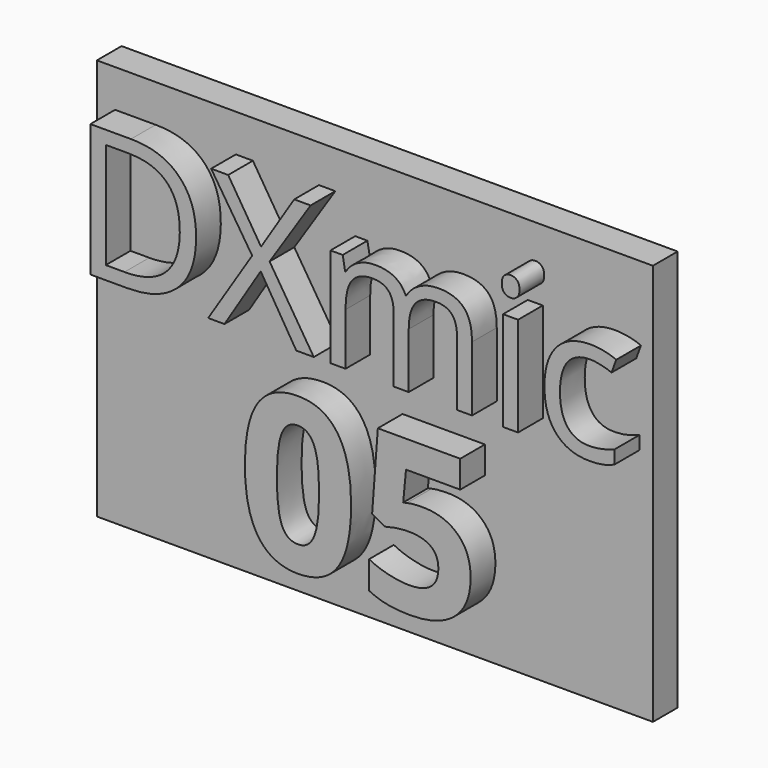
from build123d import *

# Parameters (mm, degrees)
F0_W           = 36
F0_H           = 26
F0_W_2         = 0.9740889422
F0_H_2         = 6.4282362755
F0_TEXT_SIZE   = 13.7795519549
F0_TEXT_SIZE_2 = 12.0118867629
F1_DEPTH       = 2
F2_DEPTH       = 2


# Not quite as in the source:
# - Text() gives the source's letters only with a copy of the font that has no kerning and outlines rounded to 1/6400 em; it was checked with that copy


with BuildPart() as f1:
    # F0 (on Front) → F1 (new body)
    with BuildSketch(Plane.XZ):
        with Locations((-18, 13)):
            Rectangle(F0_W, F0_H)
        with BuildLine():
            add(Edge.make_bspline(
                [(-18.8107192494, 11.141487038), (-17.9398085047, 9.8496540422), (-17.9398085047, 7.3585694154)],
                knots=[0, 0, 0, 1, 1, 1], degree=2))
            add(Edge.make_bspline(
                [(-17.9398085047, 7.3585694154), (-17.9398085047, 4.7835156438), (-18.7838060619, 3.5444324953)],
                knots=[0, 0, 0, 1, 1, 1], degree=2))
            add(Edge.make_bspline(
                [(-18.7838060619, 3.5444324953), (-19.6278036192, 2.3053493469), (-21.3846964934, 2.3053493469)],
                knots=[0, 0, 0, 1, 1, 1], degree=2))
            add(Edge.make_bspline(
                [(-21.3846964934, 2.3053493469), (-23.0877629929, 2.3053493469), (-23.9522145725, 3.5842640127)],
                knots=[0, 0, 0, 1, 1, 1], degree=2))
            add(Edge.make_bspline(
                [(-23.9522145725, 3.5842640127), (-24.8166661522, 4.8631786785), (-24.8166661522, 7.3585694154)],
                knots=[0, 0, 0, 1, 1, 1], degree=2))
            add(Edge.make_bspline(
                [(-24.8166661522, 7.3585694154), (-24.8166661522, 9.9637659569), (-23.97482165, 11.1985429953)],
                knots=[0, 0, 0, 1, 1, 1], degree=2))
            add(Edge.make_bspline(
                [(-23.97482165, 11.1985429953), (-23.1329771477, 12.4333200338), (-21.3846964934, 12.4333200338)],
                knots=[0, 0, 0, 1, 1, 1], degree=2))
            add(Edge.make_bspline(
                [(-21.3846964934, 12.4333200338), (-19.681629994, 12.4333200338), (-18.8107192494, 11.141487038)],
                knots=[0, 0, 0, 1, 1, 1], degree=2))
        make_face(mode=Mode.SUBTRACT)
        with BuildLine():
            add(Edge.make_bspline(
                [(-14.3334413915, 8.6310249162), (-13.9222078878, 8.7257593359), (-13.3171994348, 8.7257593359)],
                knots=[0, 0, 0, 1, 1, 1], degree=2))
            add(Edge.make_bspline(
                [(-13.3171994348, 8.7257593359), (-11.8918770295, 8.7257593359), (-11.0468029447, 7.9248228785)],
                knots=[0, 0, 0, 1, 1, 1], degree=2))
            add(Edge.make_bspline(
                [(-11.0468029447, 7.9248228785), (-10.20172886, 7.1238864211), (-10.20172886, 5.7308598407)],
                knots=[0, 0, 0, 1, 1, 1], degree=2))
            add(Edge.make_bspline(
                [(-10.20172886, 5.7308598407), (-10.20172886, 4.0837727711), (-11.2179708167, 3.194561059)],
                knots=[0, 0, 0, 1, 1, 1], degree=2))
            add(Edge.make_bspline(
                [(-11.2179708167, 3.194561059), (-12.2342127734, 2.3053493469), (-14.1245950572, 2.3053493469)],
                knots=[0, 0, 0, 1, 1, 1], degree=2))
            add(Edge.make_bspline(
                [(-14.1245950572, 2.3053493469), (-15.7673760168, 2.3053493469), (-16.7750057535, 2.8371539302)],
                knots=[0, 0, 0, 1, 1, 1], degree=2))
            Line((-16.7750057535, 2.8371539302), (-16.7750057535, 4.6349548493))
            add(Edge.make_bspline(
                [(-16.7750057535, 4.6349548493), (-16.2453542252, 4.3529046452), (-15.5380756601, 4.1742010808)],
                knots=[0, 0, 0, 1, 1, 1], degree=2))
            add(Edge.make_bspline(
                [(-15.5380756601, 4.1742010808), (-14.8307970949, 3.9954975164), (-14.1999519819, 3.9954975164)],
                knots=[0, 0, 0, 1, 1, 1], degree=2))
            add(Edge.make_bspline(
                [(-14.1999519819, 3.9954975164), (-12.2944983132, 3.9954975164), (-12.2944983132, 5.5564623863)],
                knots=[0, 0, 0, 1, 1, 1], degree=2))
            add(Edge.make_bspline(
                [(-12.2944983132, 5.5564623863), (-12.2944983132, 7.0442233864), (-14.2666966867, 7.0442233864)],
                knots=[0, 0, 0, 1, 1, 1], degree=2))
            add(Edge.make_bspline(
                [(-14.2666966867, 7.0442233864), (-14.6219507606, 7.0442233864), (-15.0525617591, 6.9731725716)],
                knots=[0, 0, 0, 1, 1, 1], degree=2))
            add(Edge.make_bspline(
                [(-15.0525617591, 6.9731725716), (-15.4831727577, 6.9021217569), (-15.7523046319, 6.8203056671)],
                knots=[0, 0, 0, 1, 1, 1], degree=2))
            Line((-15.7523046319, 6.8203056671), (-16.5812308041, 7.2659880507))
            Line((-16.5812308041, 7.2659880507), (-16.2109053454, 12.2783000743))
            Line((-16.2109053454, 12.2783000743), (-10.8756350728, 12.2783000743))
            Line((-10.8756350728, 12.2783000743), (-10.8756350728, 10.5149480351))
            Line((-10.8756350728, 10.5149480351), (-14.3872677663, 10.5149480351))
            Line((-14.3872677663, 10.5149480351), (-14.5681243857, 8.5836577064))
            Line((-14.5681243857, 8.5836577064), (-14.3334413915, 8.6310249162))
        make_face(mode=Mode.SUBTRACT)
        with BuildLine():
            add(Edge.make_bspline(
                [(-29.0847192534, 22.4564020512), (-27.9764350138, 21.3481178116), (-27.9764350138, 19.3586490665)],
                knots=[0, 0, 0, 1, 1, 1], degree=2))
            add(Edge.make_bspline(
                [(-27.9764350138, 19.3586490665), (-27.9764350138, 17.2359234526), (-29.1288254001, 16.1126243545)],
                knots=[0, 0, 0, 1, 1, 1], degree=2))
            add(Edge.make_bspline(
                [(-29.1288254001, 16.1126243545), (-30.2812157865, 14.9893252565), (-32.4452322611, 14.9893252565)],
                knots=[0, 0, 0, 1, 1, 1], degree=2))
            Line((-32.4452322611, 14.9893252565), (-34.8213336114, 14.9893252565))
            Line((-34.8213336114, 14.9893252565), (-34.8213336114, 23.5646862908))
            Line((-34.8213336114, 23.5646862908), (-32.193733382, 23.5646862908))
            add(Edge.make_bspline(
                [(-32.193733382, 23.5646862908), (-30.193003493, 23.5646862908), (-29.0847192534, 22.4564020512)],
                knots=[0, 0, 0, 1, 1, 1], degree=2))
        make_face(mode=Mode.SUBTRACT)
        Polygon((-23.2186017413, 19.5050439364), (-20.3563943486, 14.9893252565), (-21.4881393045, 14.9893252565), (-23.7929200772, 18.7599315857), (-26.1389917105, 14.9893252565), (-27.1956623742, 14.9893252565), (-24.3447161253, 19.4712605049), (-27.0023460716, 23.5646862908), (-25.8987539753, 23.5646862908), (-23.7703977895, 20.1675745657), (-21.6232730306, 23.5646862908), (-20.5628486523, 23.5646862908), align=None, mode=Mode.SUBTRACT)
        with BuildLine():
            Line((-10.1106303112, 14.9893252565), (-11.0828423961, 14.9893252565))
            Line((-11.0828423961, 14.9893252565), (-11.0828423961, 19.1709633358))
            add(Edge.make_bspline(
                [(-11.0828423961, 19.1709633358), (-11.0828423961, 19.9404748316), (-11.4112924248, 20.3242921508)],
                knots=[0, 0, 0, 1, 1, 1], degree=2))
            add(Edge.make_bspline(
                [(-11.4112924248, 20.3242921508), (-11.7397424535, 20.70810947), (-12.4323027996, 20.70810947)],
                knots=[0, 0, 0, 1, 1, 1], degree=2))
            add(Edge.make_bspline(
                [(-12.4323027996, 20.70810947), (-13.3407017361, 20.70810947), (-13.7751942026, 20.1863431388)],
                knots=[0, 0, 0, 1, 1, 1], degree=2))
            add(Edge.make_bspline(
                [(-13.7751942026, 20.1863431388), (-14.2096866691, 19.6645768075), (-14.2096866691, 18.5797532842)],
                knots=[0, 0, 0, 1, 1, 1], degree=2))
            Line((-14.2096866691, 18.5797532842), (-14.2096866691, 14.9893252565))
            Line((-14.2096866691, 14.9893252565), (-15.1837756113, 14.9893252565))
            Line((-15.1837756113, 14.9893252565), (-15.1837756113, 19.1709633358))
            add(Edge.make_bspline(
                [(-15.1837756113, 19.1709633358), (-15.1837756113, 19.9404748316), (-15.51222564, 20.3242921508)],
                knots=[0, 0, 0, 1, 1, 1], degree=2))
            add(Edge.make_bspline(
                [(-15.51222564, 20.3242921508), (-15.8406756686, 20.70810947), (-16.5388665867, 20.70810947)],
                knots=[0, 0, 0, 1, 1, 1], degree=2))
            add(Edge.make_bspline(
                [(-16.5388665867, 20.70810947), (-17.4528960951, 20.70810947), (-17.8780042751, 20.1600671365)],
                knots=[0, 0, 0, 1, 1, 1], degree=2))
            add(Edge.make_bspline(
                [(-17.8780042751, 20.1600671365), (-18.303112455, 19.6120248029), (-18.303112455, 18.3620378366)],
                knots=[0, 0, 0, 1, 1, 1], degree=2))
            Line((-18.303112455, 18.3620378366), (-18.303112455, 14.9893252565))
            Line((-18.303112455, 14.9893252565), (-19.2772013972, 14.9893252565))
            Line((-19.2772013972, 14.9893252565), (-19.2772013972, 21.417561532))
            Line((-19.2772013972, 21.417561532), (-18.4851676138, 21.417561532))
            Line((-18.4851676138, 21.417561532), (-18.3275116, 20.5373154551))
            Line((-18.3275116, 20.5373154551), (-18.2805901674, 20.5373154551))
            add(Edge.make_bspline(
                [(-18.2805901674, 20.5373154551), (-18.0046921433, 21.0065297818), (-17.5026328137, 21.271166662)],
                knots=[0, 0, 0, 1, 1, 1], degree=2))
            add(Edge.make_bspline(
                [(-17.5026328137, 21.271166662), (-17.0005734842, 21.5358035423), (-16.3793337157, 21.5358035423)],
                knots=[0, 0, 0, 1, 1, 1], degree=2))
            add(Edge.make_bspline(
                [(-16.3793337157, 21.5358035423), (-14.8722172984, 21.5358035423), (-14.4086335436, 20.4434725898)],
                knots=[0, 0, 0, 1, 1, 1], degree=2))
            Line((-14.4086335436, 20.4434725898), (-14.3617121109, 20.4434725898))
            add(Edge.make_bspline(
                [(-14.3617121109, 20.4434725898), (-14.074552943, 20.9483472053), (-13.5293258954, 21.2420753738)],
                knots=[0, 0, 0, 1, 1, 1], degree=2))
            add(Edge.make_bspline(
                [(-13.5293258954, 21.2420753738), (-12.9840988478, 21.5358035423), (-12.2859079297, 21.5358035423)],
                knots=[0, 0, 0, 1, 1, 1], degree=2))
            add(Edge.make_bspline(
                [(-12.2859079297, 21.5358035423), (-11.1954538345, 21.5358035423), (-10.6530420729, 20.9755616362)],
                knots=[0, 0, 0, 1, 1, 1], degree=2))
            add(Edge.make_bspline(
                [(-10.6530420729, 20.9755616362), (-10.1106303112, 20.4153197302), (-10.1106303112, 19.1822244797)],
                knots=[0, 0, 0, 1, 1, 1], degree=2))
            Line((-10.1106303112, 19.1822244797), (-10.1106303112, 14.9893252565))
        make_face(mode=Mode.SUBTRACT)
        with Locations((-7.6172253793, 18.2034433942)):
            Rectangle(F0_W_2, F0_H_2, mode=Mode.SUBTRACT)
        with BuildLine():
            add(Edge.make_bspline(
                [(-0.8727386476, 15.2070407041), (-1.5165007038, 14.8710832462), (-2.4962202179, 14.8710832462)],
                knots=[0, 0, 0, 1, 1, 1], degree=2))
            add(Edge.make_bspline(
                [(-2.4962202179, 14.8710832462), (-3.8926020541, 14.8710832462), (-4.6583598353, 15.7306838926)],
                knots=[0, 0, 0, 1, 1, 1], degree=2))
            add(Edge.make_bspline(
                [(-4.6583598353, 15.7306838926), (-5.4241176164, 16.5902845391), (-5.4241176164, 18.1630909621)],
                knots=[0, 0, 0, 1, 1, 1], degree=2))
            add(Edge.make_bspline(
                [(-5.4241176164, 18.1630909621), (-5.4241176164, 19.7753113886), (-4.6461602628, 20.6555574654)],
                knots=[0, 0, 0, 1, 1, 1], degree=2))
            add(Edge.make_bspline(
                [(-4.6461602628, 20.6555574654), (-3.8682029091, 21.5358035423), (-2.4324070695, 21.5358035423)],
                knots=[0, 0, 0, 1, 1, 1], degree=2))
            add(Edge.make_bspline(
                [(-2.4324070695, 21.5358035423), (-1.9688233147, 21.5358035423), (-1.50523956, 21.4353916764)],
                knots=[0, 0, 0, 1, 1, 1], degree=2))
            add(Edge.make_bspline(
                [(-1.50523956, 21.4353916764), (-1.0416558052, 21.3349798105), (-0.7788957823, 21.1998460844)],
                knots=[0, 0, 0, 1, 1, 1], degree=2))
            Line((-0.7788957823, 21.1998460844), (-1.0773160941, 20.3740288694))
            add(Edge.make_bspline(
                [(-1.0773160941, 20.3740288694), (-1.4001355508, 20.5035320236), (-1.7811375841, 20.5879906024)],
                knots=[0, 0, 0, 1, 1, 1], degree=2))
            add(Edge.make_bspline(
                [(-1.7811375841, 20.5879906024), (-2.1621396173, 20.6724491812), (-2.4549293572, 20.6724491812)],
                knots=[0, 0, 0, 1, 1, 1], degree=2))
            add(Edge.make_bspline(
                [(-2.4549293572, 20.6724491812), (-4.4143683854, 20.6724491812), (-4.4143683854, 18.174352106)],
                knots=[0, 0, 0, 1, 1, 1], degree=2))
            add(Edge.make_bspline(
                [(-4.4143683854, 18.174352106), (-4.4143683854, 16.9900551454), (-3.9367082008, 16.3566158044)],
                knots=[0, 0, 0, 1, 1, 1], degree=2))
            add(Edge.make_bspline(
                [(-3.9367082008, 16.3566158044), (-3.4590480163, 15.7231764634), (-2.5206193629, 15.7231764634)],
                knots=[0, 0, 0, 1, 1, 1], degree=2))
            add(Edge.make_bspline(
                [(-2.5206193629, 15.7231764634), (-1.7173244356, 15.7231764634), (-0.8727386476, 16.0685182078)],
                knots=[0, 0, 0, 1, 1, 1], degree=2))
            Line((-0.8727386476, 16.0685182078), (-0.8727386476, 15.2070407041))
        make_face(mode=Mode.SUBTRACT)
        with BuildLine():
            add(Edge.make_bspline(
                [(-8.0226265575, 22.6694253555), (-8.1868515719, 22.8308350839), (-8.1868515719, 23.1592851126)],
                knots=[0, 0, 0, 1, 1, 1], degree=2))
            add(Edge.make_bspline(
                [(-8.1868515719, 23.1592851126), (-8.1868515719, 23.4933657132), (-8.0226265575, 23.6491448696)],
                knots=[0, 0, 0, 1, 1, 1], degree=2))
            add(Edge.make_bspline(
                [(-8.0226265575, 23.6491448696), (-7.8584015432, 23.8049240261), (-7.6106563787, 23.8049240261)],
                knots=[0, 0, 0, 1, 1, 1], degree=2))
            add(Edge.make_bspline(
                [(-7.6106563787, 23.8049240261), (-7.3760492154, 23.8049240261), (-7.2061936291, 23.6463295837)],
                knots=[0, 0, 0, 1, 1, 1], degree=2))
            add(Edge.make_bspline(
                [(-7.2061936291, 23.6463295837), (-7.0363380429, 23.4877351413), (-7.0363380429, 23.1592851126)],
                knots=[0, 0, 0, 1, 1, 1], degree=2))
            add(Edge.make_bspline(
                [(-7.0363380429, 23.1592851126), (-7.0363380429, 22.8308350839), (-7.2061936291, 22.6694253555)],
                knots=[0, 0, 0, 1, 1, 1], degree=2))
            add(Edge.make_bspline(
                [(-7.2061936291, 22.6694253555), (-7.3760492154, 22.5080156272), (-7.6106563787, 22.5080156272)],
                knots=[0, 0, 0, 1, 1, 1], degree=2))
            add(Edge.make_bspline(
                [(-7.6106563787, 22.5080156272), (-7.8584015432, 22.5080156272), (-8.0226265575, 22.6694253555)],
                knots=[0, 0, 0, 1, 1, 1], degree=2))
        make_face(mode=Mode.SUBTRACT)
        with Locations((-25.3140218556, 2.4409918115)):
            Text('05', F0_TEXT_SIZE, font='Open Sans', font_style=FontStyle.BOLD, text_align=(TextAlign.LEFT, TextAlign.BOTTOM))
        with BuildLine():
            add(Edge.make_bspline(
                [(-29.9293050414, 16.7282335511), (-29.0312288202, 17.605664342), (-29.0312288202, 19.3229887777)],
                knots=[0, 0, 0, 1, 1, 1], degree=2))
            add(Edge.make_bspline(
                [(-29.0312288202, 19.3229887777), (-29.0312288202, 21.0008992099), (-29.8729993222, 21.8511155698)],
                knots=[0, 0, 0, 1, 1, 1], degree=2))
            add(Edge.make_bspline(
                [(-29.8729993222, 21.8511155698), (-30.7147698243, 22.7013319298), (-32.3757885407, 22.7013319298)],
                knots=[0, 0, 0, 1, 1, 1], degree=2))
            Line((-32.3757885407, 22.7013319298), (-33.8247223815, 22.7013319298))
            Line((-33.8247223815, 22.7013319298), (-33.8247223815, 15.8508027603))
            Line((-33.8247223815, 15.8508027603), (-32.6103957041, 15.8508027603))
            add(Edge.make_bspline(
                [(-32.6103957041, 15.8508027603), (-30.8273812627, 15.8508027603), (-29.9293050414, 16.7282335511)],
                knots=[0, 0, 0, 1, 1, 1], degree=2))
        make_face()
        with BuildLine():
            add(Edge.make_bspline(
                [(-22.4343108025, 9.9594598469), (-22.749733359, 9.1692886645), (-22.749733359, 7.3585694154)],
                knots=[0, 0, 0, 1, 1, 1], degree=2))
            add(Edge.make_bspline(
                [(-22.749733359, 7.3585694154), (-22.749733359, 5.5500032213), (-22.437540385, 4.7662912039)],
                knots=[0, 0, 0, 1, 1, 1], degree=2))
            add(Edge.make_bspline(
                [(-22.437540385, 4.7662912039), (-22.125347411, 3.9825791864), (-21.3846964934, 3.9825791864)],
                knots=[0, 0, 0, 1, 1, 1], degree=2))
            add(Edge.make_bspline(
                [(-21.3846964934, 3.9825791864), (-20.6569639058, 3.9825791864), (-20.3340056569, 4.7759799513)],
                knots=[0, 0, 0, 1, 1, 1], degree=2))
            add(Edge.make_bspline(
                [(-20.3340056569, 4.7759799513), (-20.0110474079, 5.5693807162), (-20.0110474079, 7.3585694154)],
                knots=[0, 0, 0, 1, 1, 1], degree=2))
            add(Edge.make_bspline(
                [(-20.0110474079, 7.3585694154), (-20.0110474079, 9.1692886645), (-20.3383117669, 9.9594598469)],
                knots=[0, 0, 0, 1, 1, 1], degree=2))
            add(Edge.make_bspline(
                [(-20.3383117669, 9.9594598469), (-20.6655761258, 10.7496310293), (-21.3846964934, 10.7496310293)],
                knots=[0, 0, 0, 1, 1, 1], degree=2))
            add(Edge.make_bspline(
                [(-21.3846964934, 10.7496310293), (-22.118888246, 10.7496310293), (-22.4343108025, 9.9594598469)],
                knots=[0, 0, 0, 1, 1, 1], degree=2))
        make_face()
        with Locations((-36, 14.9893252565)):
            Text('DXmic', F0_TEXT_SIZE_2, font='Open Sans', text_align=(TextAlign.LEFT, TextAlign.BOTTOM))
    extrude(amount=-F1_DEPTH)

    # F0 (on Front) → F2 (join)
    with BuildSketch(Plane.XZ):
        with Locations((-36, 14.9893252565)):
            Text('DXmic', F0_TEXT_SIZE_2, font='Open Sans', text_align=(TextAlign.LEFT, TextAlign.BOTTOM))
        with Locations((-25.3140218556, 2.4409918115)):
            Text('05', F0_TEXT_SIZE, font='Open Sans', font_style=FontStyle.BOLD, text_align=(TextAlign.LEFT, TextAlign.BOTTOM))
    extrude(amount=F2_DEPTH)


solid = f1.part
